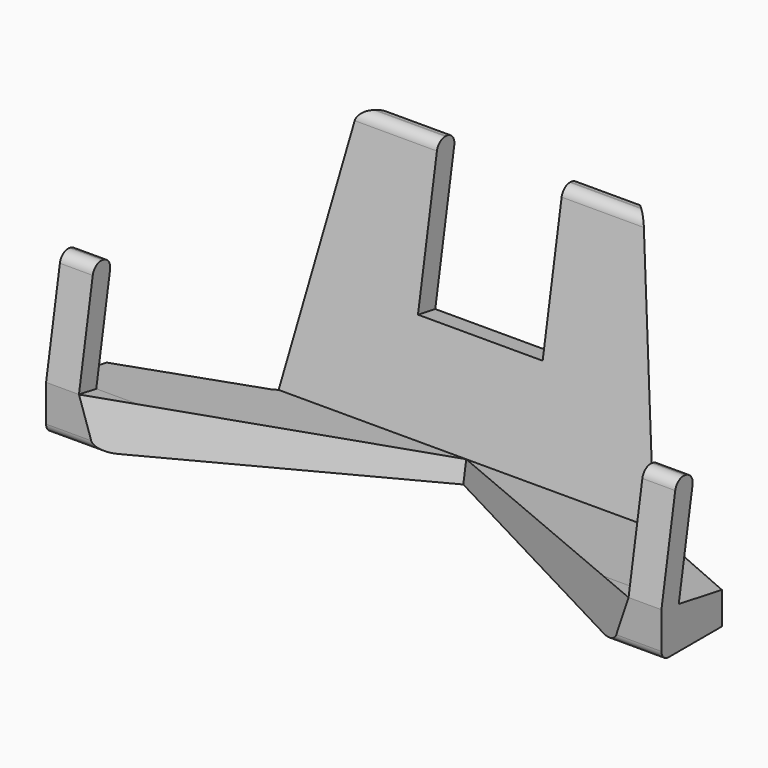
from build123d import *

# Parameters (mm, degrees)
F0_W      = 88.9
F0_H      = 38.1
F1_DEPTH  = 42.8498
F3_DEPTH  = 127
F4_W      = 79.4004
F4_H      = 15.875
F5_DEPTH  = 6.35
F7_DEPTH  = 25.4
F9_DEPTH  = 127
F10_R     = 1.524
F12_DEPTH = 25.4
F13_R     = 1.27
F14_W     = 18.0139442934
F14_H     = 19.7421588048
F14_H_2   = 6.130434971
F15_DEPTH = 25.4


with BuildPart() as f1:
    # F0 (on Front) → F1 (new body)
    with BuildSketch(Plane.XZ):
        with Locations((44.45, 19.05)):
            Rectangle(F0_W, F0_H)
    extrude(amount=F1_DEPTH)

    # F2 (on face) → F3 (cut)
    with BuildSketch(Plane(origin=(0, 0, 0), x_dir=(0, -1, 0), z_dir=(-1, 0, 0))):
        Polygon((16.8691291251, 16.8691291251), (13.1255537659, 38.1), (0, 38.1), (0, 0), (5.515703716, 0), align=None)
        Polygon((16.3495332586, 38.1), (22.5383370557, 3.0015495405), (39.7230353842, 6.0316755111), (36.9663705637, 21.6654985902), (40.0931351795, 22.2168315543), (42.8498, 6.5830084752), (42.8498, 38.1), align=None)
    extrude(amount=-F3_DEPTH, mode=Mode.SUBTRACT)

    # F4 (on face) → F5 (cut)
    with BuildSketch(Plane(origin=(0, -42.6834811822, 7.526249363), x_dir=(1, 0, 0), z_dir=(0, -0.984807753, 0.1736481777))):
        with Locations((44.45, 6.9797081012)):
            Rectangle(F4_W, F4_H)
    extrude(amount=-F5_DEPTH, mode=Mode.SUBTRACT)

    # F6 (on face) → F7 (cut)
    with BuildSketch(Plane(origin=(0, -0.1663188178, -0.9432408877), x_dir=(1, 0, 0), z_dir=(0, 0.1736481777, 0.984807753))):
        Polygon((16.7943580049, -22.7171426803), (0, -22.7171426803), (0, -31.4420426803), align=None)
        Polygon((84.1502, -43.3419426803), (44.45, -22.7171426803), (4.7498, -43.3419426803), align=None)
        Polygon((88.9, -22.7171426803), (72.1056419951, -22.7171426803), (88.9, -31.4420426803), align=None)
    extrude(amount=-F7_DEPTH, mode=Mode.SUBTRACT)

    # F8 (on face) → F9 (cut)
    with BuildSketch(Plane(origin=(0, 0, 0), x_dir=(1, 0, 0), z_dir=(0, 0, -1))):
        Polygon((35.0774, 5.515703716), (16.7943580049, 23.0675912236), (0, 23.0675912236), (0, 5.515703716), align=None)
        Polygon((72.1056419951, 23.0675912236), (53.8226, 5.515703716), (88.9, 5.515703716), (88.9, 23.0675912236), align=None)
    extrude(amount=-F9_DEPTH, mode=Mode.SUBTRACT)

    # F10
    f10_edges = [f1.edges().sort_by_distance(p)[0] for p in [
        (44.45, -13.125554, 38.1),
        (44.45, -16.349533, 38.1),
        (2.3749, -36.966371, 21.665499),
        (2.3749, -40.093135, 22.216832),
        (86.5251, -36.966371, 21.665499),
        (86.5251, -40.093135, 22.216832),
    ]]
    fillet(f10_edges, radius=F10_R)

    # F11 (on face) → F12 (cut)
    with BuildSketch(Plane(origin=(0, 0, 0), x_dir=(1, 0, 0), z_dir=(0, 0, -1))):
        Polygon((16.7943580049, 23.0675912236), (0, 31.9270868696), (0, 30.7840723544), (16.1012234683, 21.7536620769), align=None)
        Polygon((88.9, 31.9270868696), (72.1056419951, 23.0675912236), (72.6024817226, 22.125765121), (88.9, 30.4145570844), align=None)
    extrude(amount=-F12_DEPTH, mode=Mode.SUBTRACT)

    # F13
    f13_edges = [f1.edges().sort_by_distance(p)[0] for p in [
        (44.45, -5.515704, 0),
        (85.42491, -42.8498, 0),
        (3.47509, -42.8498, 0),
    ]]
    fillet(f13_edges, radius=F13_R)

    # F14 (on face) → F15 (cut)
    with BuildSketch(Plane(origin=(0, -19.245253622, 3.3934574641), x_dir=(-1, 0, 0), z_dir=(0, 0.984807753, -0.1736481777))):
        with Locations((-44.45, 23.5546350199)):
            Rectangle(F14_W, F14_H)
        with Locations((-44.45, 36.4909319078)):
            Rectangle(F14_W, F14_H_2)
    extrude(amount=-F15_DEPTH, mode=Mode.SUBTRACT)


solid = f1.part
